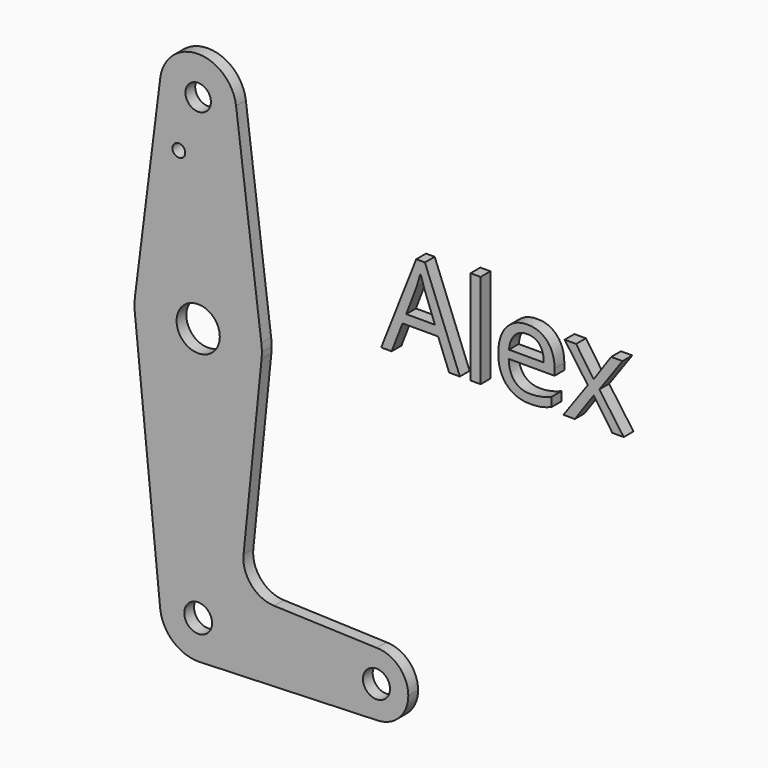
from build123d import *

# Parameters (mm, degrees)
F0_R         = 3.464105236
F0_R_2       = 5.3894449117
F0_R_3       = 3.3729933841
F0_R_4       = 1.5875
F0_R_5       = 3.175
F0_TEXT_SIZE = 30.9989942859
F1_DEPTH     = 3.048


# Not quite as in the source:
# - Text() gives the source's letters only with a copy of the font that has no kerning and outlines rounded to 1/6400 em; it was checked with that copy


with BuildPart() as f1:
    # F0 (on Front) → F1 (new body)
    with BuildSketch(Plane.XZ):
        with BuildLine():
            ThreePointArc((-27.0383486278, -33.4801347283), (-20.6767564569, -30.5017439514), (-18.0866952197, -23.9724063621))
            ThreePointArc((-18.0866952197, -23.9724063621), (-28.0882007748, -14.45933286), (-37.089019095, -24.9242241825))
            ThreePointArc((-37.089019095, -24.9242241825), (-33.9622686843, -31.0714092266), (-27.5061221152, -33.496821269))
            Line((-27.5061221152, -33.496821269), (-27.0383486278, -33.4801347283))
        make_face()
        with Locations((-27.6116952197, -23.9724063621)):
            Circle(F0_R, mode=Mode.SUBTRACT)
        with BuildLine():
            ThreePointArc((-37.089019095, -24.9242241825), (-28.0882007748, -14.45933286), (-18.0866952197, -23.9724063621))
            ThreePointArc((-18.0866952197, -23.9724063621), (-20.6767564569, -30.5017439514), (-27.0383486278, -33.4801347283))
            ThreePointArc((-27.0383486278, -33.4801347283), (-27.1548983409, -33.486446598), (-27.2715166483, -33.4913298064))
            Line((-27.2715166483, -33.4913298064), (17.1217869232, -31.9048425657))
            ThreePointArc((17.1217869232, -31.9048425657), (8.9015801854, -24.0833520913), (16.899947918, -16.035145728))
            Line((16.899947918, -16.035145728), (-8.6782722472, -15.1227654112))
            ThreePointArc((-8.6782722472, -15.1227654112), (-14.38703349, -12.4025225349), (-16.3046039996, -6.3765288762))
            Line((-16.3046039996, -6.3765288762), (-11.8174924161, 37.9279740585))
            ThreePointArc((-11.8174924161, 37.9279740585), (-27.4283601625, 23.6536523108), (-43.3647405476, 37.5636211595))
            Line((-43.3647405476, 37.5636211595), (-37.089019095, -24.9242241825))
        make_face()
        with BuildLine():
            ThreePointArc((-27.2715166483, -33.4913298064), (-27.1548983409, -33.486446598), (-27.0383486278, -33.4801347283))
            Line((-27.0383486278, -33.4801347283), (-27.5061221152, -33.496821269))
            ThreePointArc((-27.5061221152, -33.496821269), (-27.3888024693, -33.4947980691), (-27.2715166483, -33.4913298064))
        make_face()
        with BuildLine():
            Line((-43.4406792761, 38.3197489696), (-43.3647405476, 37.5636211595))
            ThreePointArc((-43.3647405476, 37.5636211595), (-27.4283601625, 23.6536523108), (-11.8174924161, 37.9279740585))
            ThreePointArc((-11.8174924161, 37.9279740585), (-11.7569073859, 38.7267642263), (-11.7366952197, 39.5275936379))
            ThreePointArc((-11.7366952197, 39.5275936379), (-11.7678537293, 40.5217323746), (-11.861206946, 41.5119686379))
            ThreePointArc((-11.861206946, 41.5119686379), (-27.6116952197, 55.4025936379), (-43.3621834934, 41.5119686379))
            ThreePointArc((-43.3621834934, 41.5119686379), (-43.481897952, 39.917837454), (-43.4406792761, 38.3197489696))
        make_face()
        with Locations((-27.6116952197, 39.5275936379)):
            Circle(F0_R_2, mode=Mode.SUBTRACT)
        with BuildLine():
            ThreePointArc((-43.4406792761, 38.3197489696), (-43.4072350118, 37.9412306039), (-43.3647405476, 37.5636211595))
            Line((-43.3647405476, 37.5636211595), (-43.4406792761, 38.3197489696))
        make_face()
        with BuildLine():
            ThreePointArc((16.899947918, -16.035145728), (8.9015801854, -24.0833520913), (17.1217869232, -31.9048425657))
            ThreePointArc((17.1217869232, -31.9048425657), (22.550311685, -29.4839291435), (24.7758047803, -23.9724063621))
            ThreePointArc((24.7758047803, -23.9724063621), (22.4727168462, -18.3815829055), (16.899947918, -16.035145728))
        make_face()
        with Locations((16.8383047803, -23.9724063621)):
            Circle(F0_R_3, mode=Mode.SUBTRACT)
        with BuildLine():
            Line((-37.0619881839, 91.5182186379), (-43.3621834934, 41.5119686379))
            ThreePointArc((-43.3621834934, 41.5119686379), (-27.6116952197, 55.4025936379), (-11.861206946, 41.5119686379))
            Line((-11.861206946, 41.5119686379), (-18.1614022555, 91.5182186379))
            ThreePointArc((-18.1614022555, 91.5182186379), (-18.1053903255, 90.9240768799), (-18.0866952197, 90.3275936379))
            ThreePointArc((-18.0866952197, 90.3275936379), (-28.2081784617, 80.8212887437), (-37.0619881839, 91.5182186379))
        make_face()
        with Locations((-32.4319377542, 77.0935565233)):
            Circle(F0_R_4, mode=Mode.SUBTRACT)
        with BuildLine():
            ThreePointArc((-18.1614022555, 91.5182186379), (-27.6116952197, 99.8525936379), (-37.0619881839, 91.5182186379))
            ThreePointArc((-37.0619881839, 91.5182186379), (-28.2081784617, 80.8212887437), (-18.0866952197, 90.3275936379))
            ThreePointArc((-18.0866952197, 90.3275936379), (-18.1053903255, 90.9240768799), (-18.1614022555, 91.5182186379))
        make_face()
        with Locations((-27.6116952197, 90.3275936379)):
            Circle(F0_R_5, mode=Mode.SUBTRACT)
        with Locations((18.0109329522, 50.2514801919)):
            Text('Alex', F0_TEXT_SIZE, font='Open Sans', text_align=(TextAlign.LEFT, TextAlign.BOTTOM))
    extrude(amount=F1_DEPTH)


solid = f1.part
